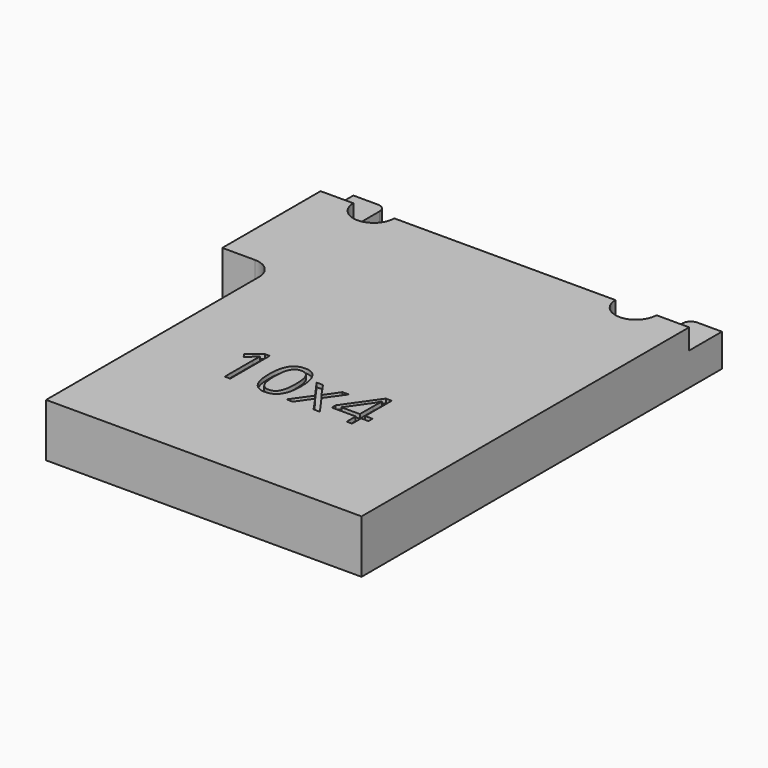
from build123d import *

# Parameters (mm, degrees)
F1_DEPTH     = 13
F2_W         = 107.3082715438
F2_H         = 14.5000026375
F3_DEPTH     = 5
F4_R         = 3
F5_DEPTH     = 10
F6_TEXT_SIZE = 16.861082986
F7_DEPTH     = 1


# Not quite as in the source:
# - Text() gives the source's letters only with a copy of the font that has no kerning and outlines rounded to 1/6400 em; it was checked with that copy


with BuildPart() as f1:
    # F0 (on Top) → F1 (new body)
    with BuildSketch(Plane.XY):
        with BuildLine():
            Line((-40.4800007343, 29.9199996144), (-40.4800007343, -10.0800003856))
            Line((-40.4800007343, -10.0800003856), (-32.5100003928, -10.0800003856))
            ThreePointArc((-32.5100003928, -10.0800003856), (-28.9744664869, -11.5444664797), (-27.5100003928, -15.0800003856))
            Line((-27.5100003928, -15.0800003856), (-27.5100003928, -80.0800003856))
            Line((-27.5100003928, -80.0800003856), (49.5199992657, -80.0800003856))
            Line((49.5199992657, -80.0800003856), (49.5199992657, 29.9199996144))
            Line((49.5199992657, 29.9199996144), (43.5199992657, 29.9199996144))
            ThreePointArc((43.5199992657, 29.9199996144), (42.1057857033, 29.3342131767), (41.5199992657, 27.9199996144))
            Line((41.5199992657, 27.9199996144), (41.5199992657, 19.9199996144))
            ThreePointArc((41.5199992657, 19.9199996144), (36.5199992657, 14.9199996144), (31.5199992657, 19.9199996144))
            Line((31.5199992657, 19.9199996144), (-22.4800007343, 19.9199996144))
            ThreePointArc((-22.4800007343, 19.9199996144), (-27.4800007343, 14.9199996144), (-32.4800007343, 19.9199996144))
            Line((-32.4800007343, 19.9199996144), (-32.4800007343, 27.9199996144))
            ThreePointArc((-32.4800007343, 27.9199996144), (-33.065787172, 29.3342131767), (-34.4800007343, 29.9199996144))
            Line((-34.4800007343, 29.9199996144), (-40.4800007343, 29.9199996144))
        make_face()
    extrude(amount=F1_DEPTH)

    # F2 (on face) → F3 (cut)
    with BuildSketch(Plane.XY.offset(13)):
        with Locations((10.5722389322, 27.1700009331)):
            Rectangle(F2_W, F2_H)
    extrude(amount=-F3_DEPTH, mode=Mode.SUBTRACT)

    # F4 (on face) → F5 (cut)
    with BuildSketch(Plane(origin=(0, 19.9199996144, 0), x_dir=(-1, 0, 0), z_dir=(0, 1, 0))):
        with Locations((12.4800007343, 6.5)):
            Circle(F4_R)
    extrude(amount=-F5_DEPTH, mode=Mode.SUBTRACT)

    # F6 (on face) → F7 (cut)
    with BuildSketch(Plane.XY.offset(13)):
        with Locations((-11.4510091371, -51.300637424)):
            Text('10x4', F6_TEXT_SIZE, font='Open Sans', text_align=(TextAlign.LEFT, TextAlign.BOTTOM))
    extrude(amount=-F7_DEPTH, mode=Mode.SUBTRACT)


solid = f1.part
